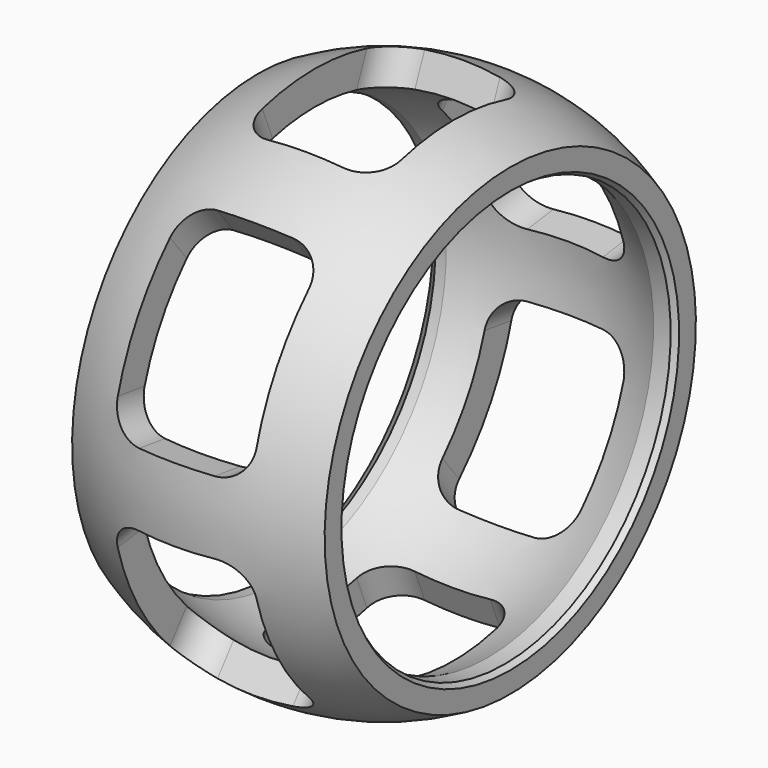
from build123d import *

# Parameters (mm, degrees)
F3_DEPTH        = 8.75
F3_COPIES_COUNT = 6
F4_R            = 4


# Not quite as in the source:
# - a pattern or mirror of a feature is missing from the dataset's text; its kind, count and spacing are read off the source's solid


with BuildPart() as f1:
    # F0 (on Front) → F1 (revolve)
    with BuildSketch(Plane.XZ):
        with BuildLine():
            Line((-15.9162652654, 29.25), (-15.9162652654, 27.65))
            Line((-15.9162652654, 27.65), (-14.4162652654, 26.15))
            Line((-14.4162652654, 26.15), (-13.0662652654, 26.15))
            ThreePointArc((-13.0662652654, 26.15), (0, 29.2326835577), (13.0662652654, 26.15))
            Line((13.0662652654, 26.15), (15.2162652654, 26.15))
            Line((15.2162652654, 26.15), (15.9162652654, 26.6))
            Line((15.9162652654, 26.6), (15.9162652654, 29.25))
            ThreePointArc((15.9162652654, 29.25), (0, 33.3), (-15.9162652654, 29.25))
        make_face()
    revolve(axis=Axis((0, 0, 0), (1, 0, 0)))

    # F2 (on Right) → F3 (cut, symmetric)
    with BuildSketch(Plane.YZ):
        Polygon((-13.7368916784, 34), (-9.69662942, 24), (0, 24), (9.69662942, 24), (13.7368916784, 34), align=None)
    f3 = extrude(amount=F3_DEPTH, both=True, mode=Mode.SUBTRACT)

    # F3_copies: F3 ×6 about axis
    f3_copies_axis = Axis((0, 0, 0), (1, 0, 0))
    for i in range(1, F3_COPIES_COUNT):
        add(f3.rotate(f3_copies_axis, i * 360 / F3_COPIES_COUNT), mode=Mode.SUBTRACT)

    # F4
    f4_edges = [f1.edges().sort_by_distance(p)[0] for p in [
        (-8.75, -11.24237, 27.825843),
        (8.75, -11.24237, 27.825843),
        (8.75, 11.24237, 27.825843),
        (-8.75, 11.24237, 27.825843),
        (8.75, -18.476702, 23.6491),
        (-8.75, -18.476702, 23.6491),
        (-8.75, -29.719072, 4.176743),
        (8.75, -29.719072, 4.176743),
        (8.75, -29.719072, -4.176743),
        (-8.75, -29.719072, -4.176743),
        (-8.75, -18.476702, -23.6491),
        (8.75, -18.476702, -23.6491),
        (8.75, -11.24237, -27.825843),
        (-8.75, -11.24237, -27.825843),
        (-8.75, 11.24237, -27.825843),
        (8.75, 11.24237, -27.825843),
        (8.75, 18.476702, -23.6491),
        (-8.75, 18.476702, -23.6491),
        (-8.75, 29.719072, -4.176743),
        (8.75, 29.719072, -4.176743),
        (8.75, 29.719072, 4.176743),
        (-8.75, 29.719072, 4.176743),
        (8.75, 18.476702, 23.6491),
        (-8.75, 18.476702, 23.6491),
    ]]
    fillet(f4_edges, radius=F4_R)


solid = f1.part
